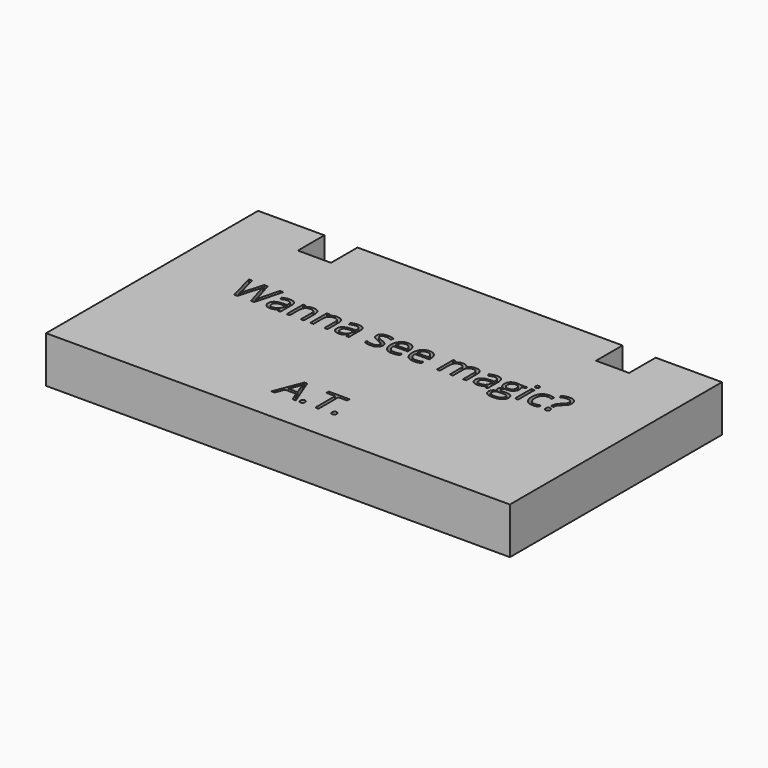
from build123d import *

# Parameters (mm, degrees)
F0_W           = 70
F0_H           = 40
F1_DEPTH       = 7
F2_W           = 5
F2_H           = 7
F3_DEPTH       = 5
F4_TEXT_SIZE   = 5.8037252662
F4_TEXT_SIZE_2 = 5.8516960775
F5_DEPTH       = 1


# Not quite as in the source:
# - Text() gives the source's letters only with a copy of the font that has no kerning and outlines rounded to 1/6400 em; it was checked with that copy


with BuildPart() as f1:
    # F0 (on Top) → F1 (new body)
    with BuildSketch(Plane.XY):
        with Locations((3.6068717018, -3.5363827487)):
            Rectangle(F0_W, F0_H)
    extrude(amount=F1_DEPTH)

    # F2 (on face) → F3 (cut)
    with BuildSketch(Plane(origin=(0, 16.4636172513, 0), x_dir=(-1, 0, 0), z_dir=(0, 1, 0))):
        with Locations((-26.1068717018, 3.5)):
            Rectangle(F2_W, F2_H)
        with Locations((18.8931282982, 3.5)):
            Rectangle(F2_W, F2_H)
    extrude(amount=-F3_DEPTH, mode=Mode.SUBTRACT)

    # F4 (on face) → F5 (cut)
    with BuildSketch(Plane.XY.offset(7)):
        with Locations((-21.3931282982, -2.0180078456)):
            Text('Wanna see magic?', F4_TEXT_SIZE, font='Open Sans', text_align=(TextAlign.LEFT, TextAlign.BOTTOM))
        with Locations((-1.3931282982, -18.5363827487)):
            Text('A.T.', F4_TEXT_SIZE_2, font='Open Sans', text_align=(TextAlign.LEFT, TextAlign.BOTTOM))
    extrude(amount=-F5_DEPTH, mode=Mode.SUBTRACT)


solid = f1.part
